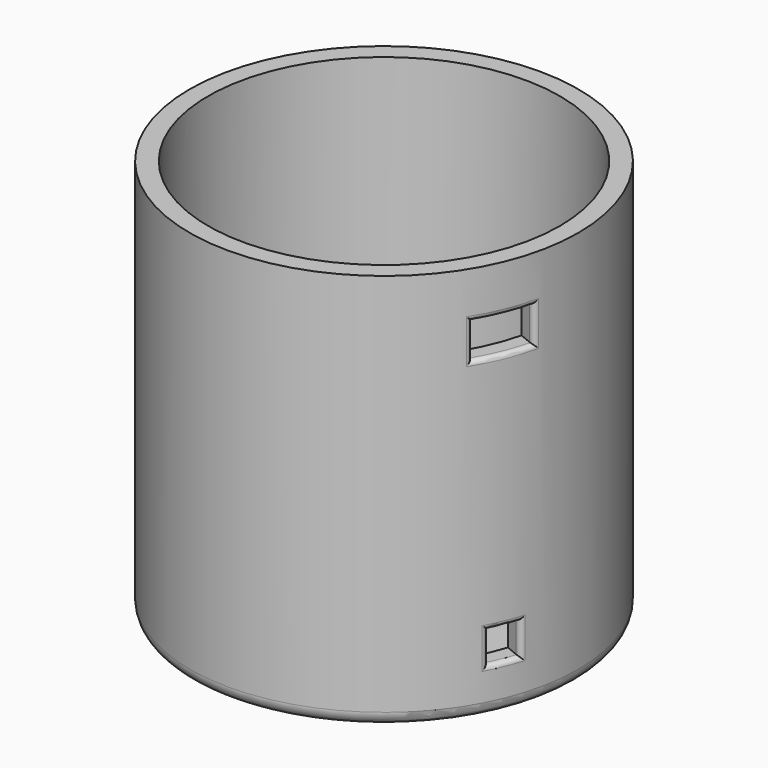
from build123d import *

# Parameters (mm, degrees)
F0_R           = 42
F0_R_2         = 38
F1_DEPTH       = 86
F2_DEPTH       = 3
F7_R           = 2.625
F8_DEPTH       = 4.0917746397
F9_R           = 2.625
F10_DEPTH      = 4.0917746397
F11_R          = 3
F14_W          = 11.6
F14_H          = 7.5
F14_W_2        = 6
F14_H_2        = 6.7
F15_DEPTH      = 54.8766446555
F16_R          = 1.1
F17_DEPTH      = 10
F18_T1_DEPTH   = 7.5
F18_T3_DEPTH   = 6.7
F18_T8_ANGLE   = 22.6962930478
F18_T14_ANGLE  = 22.6962930478
F18_T20_ANGLE  = 15.0130363442
F18_T26_ANGLE  = 15.0130363442
F18_T33_DEPTH  = 10.4488940484
F18_T37_ANGLE  = 22.6962930478
F18_T44_ANGLE  = 22.6962930478
F18_T48_DEPTH  = 10.4488940484
F18_T55_DEPTH  = 10.4488940484
F18_T59_ANGLE  = 22.6962930478
F18_T66_DEPTH  = 10.4488940484
F18_T70_ANGLE  = 22.6962930478
F18_T77_ANGLE  = 15.0130363442
F18_T81_DEPTH  = 9.4537517655
F18_T88_ANGLE  = 15.0130363442
F18_T92_DEPTH  = 9.4537517655
F18_T99_ANGLE  = 15.0130363442
F18_T103_DEPTH = 9.4537517655
F18_T110_DEPTH = 9.4537517655
F18_T114_ANGLE = 15.0130363442
F19_DEPTH      = 40


# Not quite as in the source:
# - a fillet or chamfer that OpenCascade refuses, or shapes differently, is made with other operations: its cross-section is extruded or revolved along the edge and cut away or added


with BuildPart() as f1:
    # F0 (on Top) → F1 (new body)
    with BuildSketch(Plane.XY):
        Circle(F0_R)
        Circle(F0_R_2, mode=Mode.SUBTRACT)
    extrude(amount=F1_DEPTH)

    # F0 (on Top) → F2 (join)
    with BuildSketch(Plane.XY):
        Circle(F0_R)
        Circle(F0_R_2, mode=Mode.SUBTRACT)
        Circle(F0_R_2)
    extrude(amount=F2_DEPTH)

    # F7 (on plane+point) → F8 (cut, through all)
    with BuildSketch(Plane.YZ.offset(-42)):
        with Locations((0, 10)):
            Circle(F7_R)
    extrude(amount=F8_DEPTH, mode=Mode.SUBTRACT)

    # F9 (on face) → F10 (cut, through all)
    with BuildSketch(Plane(origin=(-29.6984848098, 29.6984848098, 0), x_dir=(0.7071067812, 0.7071067812, 0), z_dir=(0.7071067812, -0.7071067812, 0))):
        with Locations((0, 10)):
            Circle(F9_R)
    extrude(amount=F10_DEPTH, mode=Mode.SUBTRACT)

    # F11
    f11_edges = [f1.edges().sort_by_distance(p)[0] for p in [
        (-42, 0, 0),
    ]]
    fillet(f11_edges, radius=F11_R)

    # F14 (on face) → F15 (cut, through all)
    with BuildSketch(Plane(origin=(0, 0, 0), x_dir=(0.3826834324, 0.9238795325, 0), z_dir=(0.9238795325, -0.3826834324, 0))):
        with Locations((0, 72.25)):
            Rectangle(F14_W, F14_H)
        with Locations((0, 13.35)):
            Rectangle(F14_W_2, F14_H_2)
    extrude(amount=F15_DEPTH, mode=Mode.SUBTRACT)

    # F16 (on face) → F17 (join)
    with BuildSketch(Plane.XY.offset(3)):
        with Locations((19.5800699423, 26.6344591071)):
            Circle(F16_R)
        with Locations((2.8950722912, -13.6466885104)):
            Circle(F16_R)
        with Locations((-16.2292340318, -5.7251414605)):
            Circle(F16_R)
        with Locations((0.4557636193, 34.556006157)):
            Circle(F16_R)
    extrude(amount=F17_DEPTH)

    # F18: fillet of radius 1 on 8 edges, made by hand

    # F18_s2 → F18_t1 (cut)
    with BuildSketch(Plane.XY.offset(68.5)):
        with BuildLine():
            ThreePointArc((35.5998174413, -22.2857128706), (35.7047230458, -21.4506255904), (35.1348861726, -20.8312211268))
            Line((35.1348861726, -20.8312211268), (36.2116037163, -21.2772121363))
            ThreePointArc((36.2116037163, -21.2772121363), (35.9092511841, -21.783610339), (35.5998174413, -22.2857128706))
        make_face()
        with BuildLine():
            ThreePointArc((40.9312510161, -9.4144936274), (40.4149346017, -10.0791689704), (39.5740139881, -10.1142185497))
            Line((39.5740139881, -10.1142185497), (40.6507315318, -10.5602095591))
            ThreePointArc((40.6507315318, -10.5602095591), (40.795013609, -9.9883364302), (40.9312510161, -9.4144936274))
        make_face()
    extrude(amount=F18_T1_DEPTH, mode=Mode.SUBTRACT)

    # F18_s4 → F18_t3 (cut)
    with BuildSketch(Plane.XY.offset(10)):
        with BuildLine():
            ThreePointArc((40.1859015546, -12.2103773999), (39.6564422799, -12.8237413852), (38.8464109423, -12.843533661))
            Line((38.8464109423, -12.843533661), (39.8518769876, -13.2600113334))
            ThreePointArc((39.8518769876, -13.2600113334), (40.0223304087, -12.7362894384), (40.1859015546, -12.2103773999))
        make_face()
        with BuildLine():
            ThreePointArc((37.0497641576, -19.781682837), (37.1090937475, -18.9735847602), (36.5503103481, -18.386810856))
            Line((36.5503103481, -18.386810856), (37.5557763934, -18.8032885285))
            ThreePointArc((37.5557763934, -18.8032885285), (37.3059778599, -19.2941446018), (37.0497641576, -19.781682837))
        make_face()
    extrude(amount=F18_T3_DEPTH, mode=Mode.SUBTRACT)


with BuildPart() as f18_tool6:
    # F18_s7 → F18_t8 (revolve)
    with BuildSketch(Plane(origin=(0, 0, 0), x_dir=(0, 0, 1), z_dir=(0.193409971, 0.9811180271, 0))):
        with BuildLine():
            ThreePointArc((67.5, 42), (68.2071067812, 41.7071067812), (68.5, 41))
            Line((68.5, 41), (68.5, 42))
            Line((68.5, 42), (67.5, 42))
        make_face()
    revolve(axis=Axis((0, 0, 68.5), (0, 0, -1)), revolution_arc=F18_T8_ANGLE)

    split(bisect_by=Plane(origin=(2.2195639077, 5.3585012886, 0), x_dir=(0, 0, 1), z_dir=(-0.3826834324, -0.9238795325, 0)), keep=Keep.TOP)

    split(bisect_by=Plane(origin=(-2.2195639077, -5.3585012886, 0), x_dir=(0, 0, 1), z_dir=(0.3826834324, 0.9238795325, 0)), keep=Keep.TOP)


with BuildPart() as f1_1:
    add(f1.part)

    # F18_t5: cut F18_tool6
    add(f18_tool6.part, mode=Mode.SUBTRACT)


with BuildPart() as f18_tool12:
    # F18_s13 → F18_t14 (revolve)
    with BuildSketch(Plane(origin=(0, 0, 0), x_dir=(0, 0, 1), z_dir=(0.193409971, 0.9811180271, 0))):
        with BuildLine():
            ThreePointArc((77, 42), (76.2928932188, 41.7071067812), (76, 41))
            Line((76, 41), (76, 42))
            Line((76, 42), (77, 42))
        make_face()
    revolve(axis=Axis((0, 0, 76), (0, 0, -1)), revolution_arc=F18_T14_ANGLE)

    split(bisect_by=Plane(origin=(2.2195639077, 5.3585012886, 0), x_dir=(0, 0, 1), z_dir=(-0.3826834324, -0.9238795325, 0)), keep=Keep.TOP)

    split(bisect_by=Plane(origin=(-2.2195639077, -5.3585012886, 0), x_dir=(0, 0, 1), z_dir=(0.3826834324, 0.9238795325, 0)), keep=Keep.TOP)


with BuildPart() as f1_2:
    add(f1_1.part)

    # F18_t11: cut F18_tool12
    add(f18_tool12.part, mode=Mode.SUBTRACT)


with BuildPart() as f18_tool18:
    # F18_s19 → F18_t20 (revolve)
    with BuildSketch(Plane(origin=(0, 0, 0), x_dir=(0, 0, 1), z_dir=(0.2587091563, 0.9659552642, 0))):
        with BuildLine():
            ThreePointArc((9, 42), (9.7071067812, 41.7071067812), (10, 41))
            Line((10, 41), (10, 42))
            Line((10, 42), (9, 42))
        make_face()
    revolve(axis=Axis((0, 0, 10), (0, 0, -1)), revolution_arc=F18_T20_ANGLE)

    split(bisect_by=Plane(origin=(1.1480502971, 2.7716385975, 0), x_dir=(0, 0, 1), z_dir=(-0.3826834324, -0.9238795325, 0)), keep=Keep.TOP)

    split(bisect_by=Plane(origin=(-1.1480502971, -2.7716385975, 0), x_dir=(0, 0, 1), z_dir=(0.3826834324, 0.9238795325, 0)), keep=Keep.TOP)


with BuildPart() as f1_3:
    add(f1_2.part)

    # F18_t17: cut F18_tool18
    add(f18_tool18.part, mode=Mode.SUBTRACT)


with BuildPart() as f18_tool24:
    # F18_s25 → F18_t26 (revolve)
    with BuildSketch(Plane(origin=(0, 0, 0), x_dir=(0, 0, 1), z_dir=(0.2587091563, 0.9659552642, 0))):
        with BuildLine():
            ThreePointArc((17.7, 42), (16.9928932188, 41.7071067812), (16.7, 41))
            Line((16.7, 41), (16.7, 42))
            Line((16.7, 42), (17.7, 42))
        make_face()
    revolve(axis=Axis((0, 0, 16.7), (0, 0, -1)), revolution_arc=F18_T26_ANGLE)

    split(bisect_by=Plane(origin=(-1.1480502971, -2.7716385975, 0), x_dir=(0, 0, 1), z_dir=(0.3826834324, 0.9238795325, 0)), keep=Keep.TOP)

    split(bisect_by=Plane(origin=(1.1480502971, 2.7716385975, 0), x_dir=(0, 0, 1), z_dir=(-0.3826834324, -0.9238795325, 0)), keep=Keep.TOP)


with BuildPart() as f1_4:
    add(f1_3.part)

    # F18_t23: cut F18_tool24
    add(f18_tool24.part, mode=Mode.SUBTRACT)


with BuildPart() as f18_tool31:
    # F18_s32 → F18_t33 (new body)
    with BuildSketch(Plane.XY.offset(76)):
        with BuildLine():
            ThreePointArc((40.9312510161, -9.4144936274), (40.4149346017, -10.0791689704), (39.5740139881, -10.1142185497))
            Line((39.5740139881, -10.1142185497), (40.6507315318, -10.5602095591))
            ThreePointArc((40.6507315318, -10.5602095591), (40.795013609, -9.9883364302), (40.9312510161, -9.4144936274))
        make_face()
    extrude(amount=-F18_T33_DEPTH)

    split(bisect_by=Plane.XY.offset(68.5), keep=Keep.BOTTOM)


with BuildPart() as f18_tool35:
    # F18_s36 → F18_t37 (revolve)
    with BuildSketch(Plane(origin=(0, 0, 0), x_dir=(0, 0, 1), z_dir=(0.193409971, 0.9811180271, 0))):
        with BuildLine():
            ThreePointArc((67.5, 42), (68.2071067812, 41.7071067812), (68.5, 41))
            Line((68.5, 41), (68.5, 42))
            Line((68.5, 42), (67.5, 42))
        make_face()
    revolve(axis=Axis((0, 0, 68.5), (0, 0, -1)), revolution_arc=F18_T37_ANGLE)

    split(bisect_by=Plane(origin=(2.2195639077, 5.3585012886, 0), x_dir=(0, 0, 1), z_dir=(0.3826834324, 0.9238795325, 0)), keep=Keep.TOP)


with BuildPart() as f18_tool31_1:
    add(f18_tool31.part)

    # F18_t39: intersect F18_tool35
    add(f18_tool35.part, mode=Mode.INTERSECT)


with BuildPart() as f1_5:
    add(f1_4.part)

    # F18_t29: cut F18_tool31
    add(f18_tool31_1.part, mode=Mode.SUBTRACT)


with BuildPart() as f18_tool42:
    # F18_s43 → F18_t44 (revolve)
    with BuildSketch(Plane(origin=(0, 0, 0), x_dir=(0, 0, 1), z_dir=(0.193409971, 0.9811180271, 0))):
        with BuildLine():
            ThreePointArc((67.5, 42), (68.2071067812, 41.7071067812), (68.5, 41))
            Line((68.5, 41), (68.5, 42))
            Line((68.5, 42), (67.5, 42))
        make_face()
    revolve(axis=Axis((0, 0, 68.5), (0, 0, -1)), revolution_arc=F18_T44_ANGLE)

    split(bisect_by=Plane(origin=(-2.2195639077, -5.3585012886, 0), x_dir=(0, 0, 1), z_dir=(-0.3826834324, -0.9238795325, 0)), keep=Keep.TOP)


with BuildPart() as f18_tool46:
    # F18_s47 → F18_t48 (new body)
    with BuildSketch(Plane.XY.offset(76)):
        with BuildLine():
            ThreePointArc((35.5998174413, -22.2857128706), (35.7047230458, -21.4506255904), (35.1348861726, -20.8312211268))
            Line((35.1348861726, -20.8312211268), (36.2116037163, -21.2772121363))
            ThreePointArc((36.2116037163, -21.2772121363), (35.9092511841, -21.783610339), (35.5998174413, -22.2857128706))
        make_face()
    extrude(amount=-F18_T48_DEPTH)

    split(bisect_by=Plane.XY.offset(68.5), keep=Keep.BOTTOM)


with BuildPart() as f18_tool42_1:
    add(f18_tool42.part)

    # F18_t50: intersect F18_tool46
    add(f18_tool46.part, mode=Mode.INTERSECT)


with BuildPart() as f1_6:
    add(f1_5.part)

    # F18_t40: cut F18_tool42
    add(f18_tool42_1.part, mode=Mode.SUBTRACT)


with BuildPart() as f18_tool53:
    # F18_s54 → F18_t55 (new body)
    with BuildSketch(Plane.XY.offset(78.9488940484)):
        with BuildLine():
            ThreePointArc((35.5998174413, -22.2857128706), (35.7047230458, -21.4506255904), (35.1348861726, -20.8312211268))
            Line((35.1348861726, -20.8312211268), (36.2116037163, -21.2772121363))
            ThreePointArc((36.2116037163, -21.2772121363), (35.9092511841, -21.783610339), (35.5998174413, -22.2857128706))
        make_face()
    extrude(amount=-F18_T55_DEPTH)

    split(bisect_by=Plane.XY.offset(76), keep=Keep.TOP)


with BuildPart() as f18_tool57:
    # F18_s58 → F18_t59 (revolve)
    with BuildSketch(Plane(origin=(0, 0, 0), x_dir=(0, 0, 1), z_dir=(0.193409971, 0.9811180271, 0))):
        with BuildLine():
            ThreePointArc((77, 42), (76.2928932188, 41.7071067812), (76, 41))
            Line((76, 41), (76, 42))
            Line((76, 42), (77, 42))
        make_face()
    revolve(axis=Axis((0, 0, 76), (0, 0, -1)), revolution_arc=F18_T59_ANGLE)

    split(bisect_by=Plane(origin=(-2.2195639077, -5.3585012886, 0), x_dir=(0, 0, 1), z_dir=(-0.3826834324, -0.9238795325, 0)), keep=Keep.TOP)


with BuildPart() as f18_tool53_1:
    add(f18_tool53.part)

    # F18_t61: intersect F18_tool57
    add(f18_tool57.part, mode=Mode.INTERSECT)


with BuildPart() as f1_7:
    add(f1_6.part)

    # F18_t51: cut F18_tool53
    add(f18_tool53_1.part, mode=Mode.SUBTRACT)


with BuildPart() as f18_tool64:
    # F18_s65 → F18_t66 (new body)
    with BuildSketch(Plane.XY.offset(78.9488940484)):
        with BuildLine():
            ThreePointArc((40.9312510161, -9.4144936274), (40.4149346017, -10.0791689704), (39.5740139881, -10.1142185497))
            Line((39.5740139881, -10.1142185497), (40.6507315318, -10.5602095591))
            ThreePointArc((40.6507315318, -10.5602095591), (40.795013609, -9.9883364302), (40.9312510161, -9.4144936274))
        make_face()
    extrude(amount=-F18_T66_DEPTH)

    split(bisect_by=Plane.XY.offset(76), keep=Keep.TOP)


with BuildPart() as f18_tool68:
    # F18_s69 → F18_t70 (revolve)
    with BuildSketch(Plane(origin=(0, 0, 0), x_dir=(0, 0, 1), z_dir=(0.193409971, 0.9811180271, 0))):
        with BuildLine():
            ThreePointArc((77, 42), (76.2928932188, 41.7071067812), (76, 41))
            Line((76, 41), (76, 42))
            Line((76, 42), (77, 42))
        make_face()
    revolve(axis=Axis((0, 0, 76), (0, 0, -1)), revolution_arc=F18_T70_ANGLE)

    split(bisect_by=Plane(origin=(2.2195639077, 5.3585012886, 0), x_dir=(0, 0, 1), z_dir=(0.3826834324, 0.9238795325, 0)), keep=Keep.TOP)


with BuildPart() as f18_tool64_1:
    add(f18_tool64.part)

    # F18_t72: intersect F18_tool68
    add(f18_tool68.part, mode=Mode.INTERSECT)


with BuildPart() as f1_8:
    add(f1_7.part)

    # F18_t62: cut F18_tool64
    add(f18_tool64_1.part, mode=Mode.SUBTRACT)


with BuildPart() as f18_tool75:
    # F18_s76 → F18_t77 (revolve)
    with BuildSketch(Plane(origin=(0, 0, 0), x_dir=(0, 0, 1), z_dir=(0.2587091563, 0.9659552642, 0))):
        with BuildLine():
            ThreePointArc((9, 42), (9.7071067812, 41.7071067812), (10, 41))
            Line((10, 41), (10, 42))
            Line((10, 42), (9, 42))
        make_face()
    revolve(axis=Axis((0, 0, 10), (0, 0, -1)), revolution_arc=F18_T77_ANGLE)

    split(bisect_by=Plane(origin=(1.1480502971, 2.7716385975, 0), x_dir=(0, 0, 1), z_dir=(0.3826834324, 0.9238795325, 0)), keep=Keep.TOP)


with BuildPart() as f18_tool79:
    # F18_s80 → F18_t81 (new body)
    with BuildSketch(Plane.XY.offset(16.7)):
        with BuildLine():
            ThreePointArc((40.1859015546, -12.2103773999), (39.6564422799, -12.8237413852), (38.8464109423, -12.843533661))
            Line((38.8464109423, -12.843533661), (39.8518769876, -13.2600113334))
            ThreePointArc((39.8518769876, -13.2600113334), (40.0223304087, -12.7362894384), (40.1859015546, -12.2103773999))
        make_face()
    extrude(amount=-F18_T81_DEPTH)

    split(bisect_by=Plane.XY.offset(10), keep=Keep.BOTTOM)


with BuildPart() as f18_tool75_1:
    add(f18_tool75.part)

    # F18_t83: intersect F18_tool79
    add(f18_tool79.part, mode=Mode.INTERSECT)


with BuildPart() as f1_9:
    add(f1_8.part)

    # F18_t73: cut F18_tool75
    add(f18_tool75_1.part, mode=Mode.SUBTRACT)


with BuildPart() as f18_tool86:
    # F18_s87 → F18_t88 (revolve)
    with BuildSketch(Plane(origin=(0, 0, 0), x_dir=(0, 0, 1), z_dir=(0.2587091563, 0.9659552642, 0))):
        with BuildLine():
            ThreePointArc((9, 42), (9.7071067812, 41.7071067812), (10, 41))
            Line((10, 41), (10, 42))
            Line((10, 42), (9, 42))
        make_face()
    revolve(axis=Axis((0, 0, 10), (0, 0, -1)), revolution_arc=F18_T88_ANGLE)

    split(bisect_by=Plane(origin=(-1.1480502971, -2.7716385975, 0), x_dir=(0, 0, 1), z_dir=(-0.3826834324, -0.9238795325, 0)), keep=Keep.TOP)


with BuildPart() as f18_tool90:
    # F18_s91 → F18_t92 (new body)
    with BuildSketch(Plane.XY.offset(16.7)):
        with BuildLine():
            ThreePointArc((37.0497641576, -19.781682837), (37.1090937475, -18.9735847602), (36.5503103481, -18.386810856))
            Line((36.5503103481, -18.386810856), (37.5557763934, -18.8032885285))
            ThreePointArc((37.5557763934, -18.8032885285), (37.3059778599, -19.2941446018), (37.0497641576, -19.781682837))
        make_face()
    extrude(amount=-F18_T92_DEPTH)

    split(bisect_by=Plane.XY.offset(10), keep=Keep.BOTTOM)


with BuildPart() as f18_tool86_1:
    add(f18_tool86.part)

    # F18_t94: intersect F18_tool90
    add(f18_tool90.part, mode=Mode.INTERSECT)


with BuildPart() as f1_10:
    add(f1_9.part)

    # F18_t84: cut F18_tool86
    add(f18_tool86_1.part, mode=Mode.SUBTRACT)


with BuildPart() as f18_tool97:
    # F18_s98 → F18_t99 (revolve)
    with BuildSketch(Plane(origin=(0, 0, 0), x_dir=(0, 0, 1), z_dir=(0.2587091563, 0.9659552642, 0))):
        with BuildLine():
            ThreePointArc((17.7, 42), (16.9928932188, 41.7071067812), (16.7, 41))
            Line((16.7, 41), (16.7, 42))
            Line((16.7, 42), (17.7, 42))
        make_face()
    revolve(axis=Axis((0, 0, 16.7), (0, 0, -1)), revolution_arc=F18_T99_ANGLE)

    split(bisect_by=Plane(origin=(1.1480502971, 2.7716385975, 0), x_dir=(0, 0, 1), z_dir=(0.3826834324, 0.9238795325, 0)), keep=Keep.TOP)


with BuildPart() as f18_tool101:
    # F18_s102 → F18_t103 (new body)
    with BuildSketch(Plane.XY.offset(19.4537517655)):
        with BuildLine():
            ThreePointArc((40.1859015546, -12.2103773999), (39.6564422799, -12.8237413852), (38.8464109423, -12.843533661))
            Line((38.8464109423, -12.843533661), (39.8518769876, -13.2600113334))
            ThreePointArc((39.8518769876, -13.2600113334), (40.0223304087, -12.7362894384), (40.1859015546, -12.2103773999))
        make_face()
    extrude(amount=-F18_T103_DEPTH)

    split(bisect_by=Plane.XY.offset(16.7), keep=Keep.TOP)


with BuildPart() as f18_tool97_1:
    add(f18_tool97.part)

    # F18_t105: intersect F18_tool101
    add(f18_tool101.part, mode=Mode.INTERSECT)


with BuildPart() as f1_11:
    add(f1_10.part)

    # F18_t95: cut F18_tool97
    add(f18_tool97_1.part, mode=Mode.SUBTRACT)


with BuildPart() as f18_tool108:
    # F18_s109 → F18_t110 (new body)
    with BuildSketch(Plane.XY.offset(19.4537517655)):
        with BuildLine():
            ThreePointArc((37.0497641576, -19.781682837), (37.1090937475, -18.9735847602), (36.5503103481, -18.386810856))
            Line((36.5503103481, -18.386810856), (37.5557763934, -18.8032885285))
            ThreePointArc((37.5557763934, -18.8032885285), (37.3059778599, -19.2941446018), (37.0497641576, -19.781682837))
        make_face()
    extrude(amount=-F18_T110_DEPTH)

    split(bisect_by=Plane.XY.offset(16.7), keep=Keep.TOP)


with BuildPart() as f18_tool112:
    # F18_s113 → F18_t114 (revolve)
    with BuildSketch(Plane(origin=(0, 0, 0), x_dir=(0, 0, 1), z_dir=(0.2587091563, 0.9659552642, 0))):
        with BuildLine():
            ThreePointArc((17.7, 42), (16.9928932188, 41.7071067812), (16.7, 41))
            Line((16.7, 41), (16.7, 42))
            Line((16.7, 42), (17.7, 42))
        make_face()
    revolve(axis=Axis((0, 0, 16.7), (0, 0, -1)), revolution_arc=F18_T114_ANGLE)

    split(bisect_by=Plane(origin=(-1.1480502971, -2.7716385975, 0), x_dir=(0, 0, 1), z_dir=(-0.3826834324, -0.9238795325, 0)), keep=Keep.TOP)


with BuildPart() as f18_tool108_1:
    add(f18_tool108.part)

    # F18_t116: intersect F18_tool112
    add(f18_tool112.part, mode=Mode.INTERSECT)


with BuildPart() as f1_12:
    add(f1_11.part)

    # F18_t106: cut F18_tool108
    add(f18_tool108_1.part, mode=Mode.SUBTRACT)

    # F14 (on face) → F19 (cut)
    with BuildSketch(Plane(origin=(0, 0, 0), x_dir=(0.3826834324, 0.9238795325, 0), z_dir=(0.9238795325, -0.3826834324, 0))):
        Polygon((-3, 16.7), (3, 16.7), (5, 16.7), (5, 31.7), (-5, 31.7), (-5, 16.7), align=None)
    extrude(amount=F19_DEPTH, mode=Mode.SUBTRACT)


solid = f1_12.part
